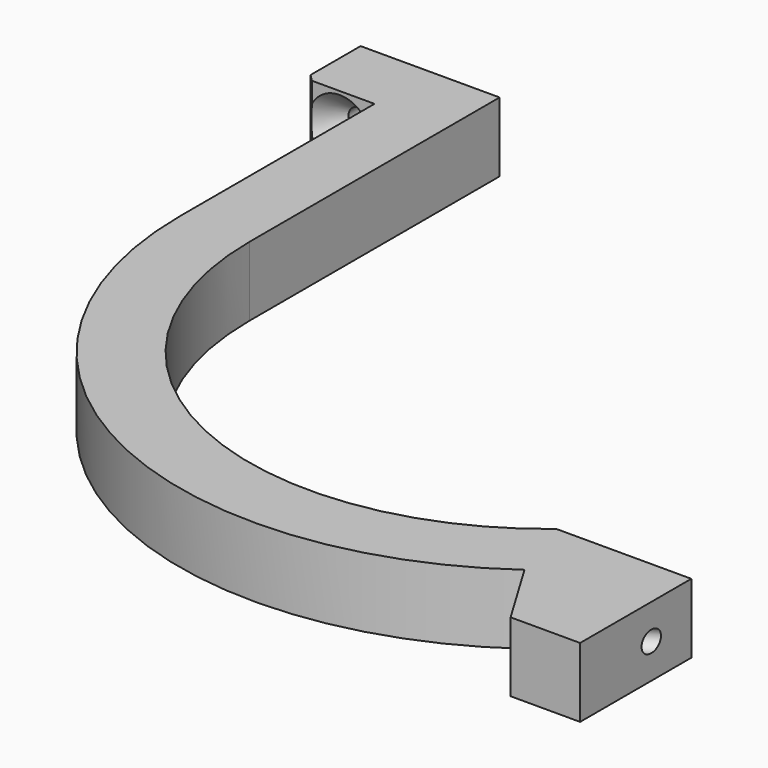
from build123d import *

# Parameters (mm, degrees)
F0_W                 = 10
F0_H                 = 10
F1_DEPTH             = 10
F4_D                 = 3
F4_CSINK_D           = 9
F4_CSINK_ANGLE       = 82
F4_ON_F2_D           = 3
F4_ON_F2_CSINK_D     = 9
F4_ON_F2_CSINK_ANGLE = 82
F5_T1_DEPTH          = 15.1433659759


# Not quite as in the source:
# - a fillet or chamfer that OpenCascade refuses, or shapes differently, is made with other operations: its cross-section is extruded or revolved along the edge and cut away or added


with BuildPart() as f1:
    # F0 (on Top) → F1 (new body)
    with BuildSketch(Plane.XY):
        with BuildLine():
            ThreePointArc((27.5680975042, -33), (-18.2149911792, -38.9514325326), (-43, 0))
            Line((-43, 0), (-43, 45))
            Line((-43, 45), (-53, 45))
            Line((-53, 45), (-53, 35))
            Line((-53, 35), (-53, 0))
            ThreePointArc((-53, 0), (-24.154244567, -47.1759734335), (30.9838667697, -43))
            Line((30.9838667697, -43), (36.9838667697, -53))
            Line((36.9838667697, -53), (46.9838667697, -53))
            Line((46.9838667697, -53), (46.9838667697, -43))
            Line((46.9838667697, -43), (46.9838667697, -33))
            Line((46.9838667697, -33), (27.5680975042, -33))
        make_face()
        with Locations((-58, 40)):
            Rectangle(F0_W, F0_H)
    extrude(amount=F1_DEPTH)

    # F4 (through all)
    with Locations(Plane(origin=(3.8116667424, 2.2870000454, 0), x_dir=(0.5144957554, -0.8574929257, 0), z_dir=(-0.8574929257, -0.5144957554, 0))):
        with Locations((58.6442156402, 5)):
            CounterSinkHole(F4_D / 2, F4_CSINK_D / 2, counter_sink_angle=F4_CSINK_ANGLE)

    # F4 on F2 (through all)
    with Locations(Plane.XZ.offset(-35)):
        with Locations((-58, 5)):
            CounterSinkHole(F4_ON_F2_D / 2, F4_ON_F2_CSINK_D / 2, counter_sink_angle=F4_ON_F2_CSINK_ANGLE)

    # F5: chamfer of 1 on 1 edges, made by hand

    # F5_s2 → F5_t1 (cut)
    with BuildSketch(Plane.XY.offset(-2.571682988)):
        Polygon((-63, 36), (-62, 35), (-63, 35), align=None)
    extrude(amount=F5_T1_DEPTH, mode=Mode.SUBTRACT)


solid = f1.part
